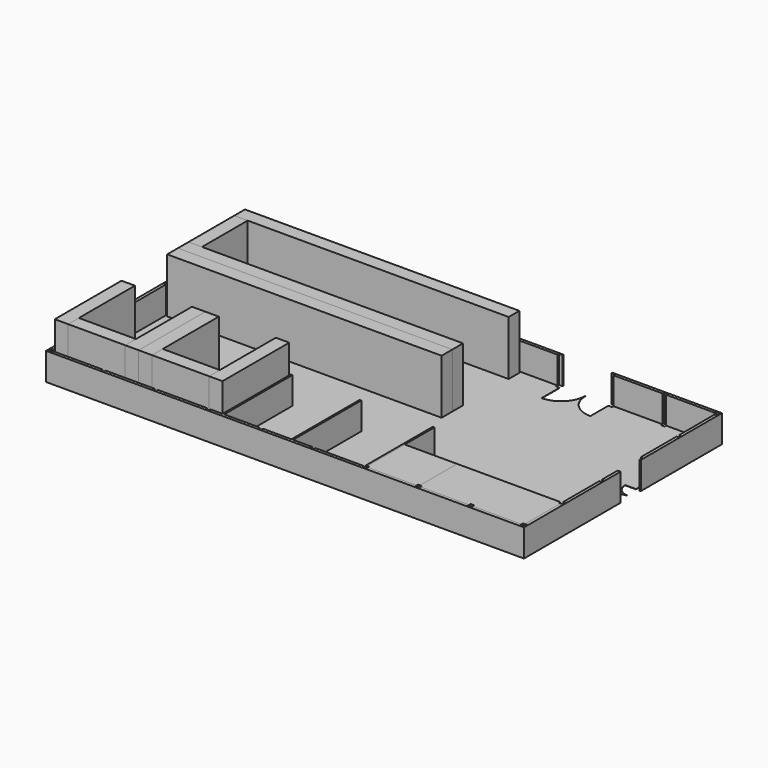
from build123d import *

# Parameters (mm, degrees)
F0_R     = 2342.0075
F0_W     = 6500
F0_H     = 150
F0_W_2   = 6127.2340836304
F1_DEPTH = 25
F2_DEPTH = 5000
F3_DEPTH = 5000
F4_DEPTH = 5000
F0_W_3   = 150
F0_H_2   = 7620
F5_DEPTH = 2500
F6_DEPTH = 2500
F7_DEPTH = 2500
F8_DEPTH = 1000
F0_H_3   = 270
F9_DEPTH = 2500


with BuildPart() as f1:
    # F0 (on Top) → F1 (new body)
    with BuildSketch(Plane.XY):
        with BuildLine():
            ThreePointArc((33274.4446, 19781.1111), (31705.4532121104, 20431.0086121104), (31055.5557, 22000))
            ThreePointArc((31055.5557, 22000), (30405.6581878896, 20431.0086121104), (28836.6668, 19781.1111))
            Line((28836.6668, 19781.1111), (28836.6668, 21830))
            Line((28836.6668, 21830), (28496.6668, 21830))
            Line((28496.6668, 21830), (28496.6668, 22000))
            Line((28496.6668, 22000), (24058.889, 22000))
            Line((24058.889, 22000), (24058.889, 21830))
            Line((24058.889, 21830), (25170, 21830))
            Line((25170, 21830), (25170, 20610))
            Line((25170, 20610), (1390, 20610))
            Line((1390, 20610), (1390, 15410))
            Line((1390, 15410), (25170, 15410))
            Line((25170, 15410), (25170, 14190))
            Line((25170, 14190), (25170, 12970))
            Line((25170, 12970), (170, 12970))
            Line((170, 12970), (170, 13030))
            Line((170, 13030), (0, 13030))
            Line((0, 13030), (0, 11370))
            Line((0, 11370), (0, 9370))
            Line((0, 9370), (0, 8970))
            Line((0, 8970), (170, 8970))
            Line((170, 8970), (170, 8630))
            Line((170, 8630), (0, 8630))
            Line((0, 8630), (0, 4570))
            Line((0, 4570), (170, 4570))
            Line((170, 4570), (170, 7770))
            Line((170, 7770), (1390, 7770))
            Line((1390, 7770), (1390, 1390))
            Line((1390, 1390), (6590, 1390))
            Line((6590, 1390), (6590, 7770))
            Line((6590, 7770), (7810, 7770))
            Line((7810, 7770), (9030, 7770))
            Line((9030, 7770), (9030, 1390))
            Line((9030, 1390), (14230, 1390))
            Line((14230, 1390), (14230, 7770))
            Line((14230, 7770), (15450, 7770))
            Line((15450, 7770), (15450, 170))
            Line((15450, 170), (14503.3334, 170))
            Line((14503.3334, 170), (14503.3334, 0))
            Line((14503.3334, 0), (15589.4327163696, 0))
            Line((15589.4327163696, 0), (15589.4327163696, 7620))
            Line((15589.4327163696, 7620), (15589.4327163696, 7770))
            Line((15589.4327163696, 7770), (15739.4327163696, 7770))
            Line((15739.4327163696, 7770), (21866.6668, 7770))
            Line((21866.6668, 7770), (22016.6668, 7770))
            Line((22016.6668, 7770), (28516.6668, 7770))
            Line((28516.6668, 7770), (28666.6668, 7770))
            Line((28666.6668, 7770), (28666.6668, 7620))
            Line((28666.6668, 7620), (28666.6668, 4400))
            Line((28666.6668, 4400), (33444.4446, 4400))
            Line((33444.4446, 4400), (42830, 4400))
            Line((42830, 4400), (42830, 4570))
            Line((42830, 4570), (43000, 4570))
            Line((43000, 4570), (43000, 8630))
            Line((43000, 8630), (42830, 8630))
            Line((42830, 8630), (42830, 8970))
            Line((42830, 8970), (43000, 8970))
            Line((43000, 8970), (43000, 10730))
            Line((43000, 10730), (41850, 10730))
            ThreePointArc((41850, 10730), (42186.8272016355, 11543.1727983645), (43000, 11880))
            ThreePointArc((43000, 11880), (42186.8272016355, 12216.8272016355), (41850, 13030))
            Line((41850, 13030), (42830, 13030))
            Line((42830, 13030), (42830, 13370))
            Line((42830, 13370), (43000, 13370))
            Line((43000, 13370), (43000, 17430))
            Line((43000, 17430), (42830, 17430))
            Line((42830, 17430), (42830, 17770))
            Line((42830, 17770), (43000, 17770))
            Line((43000, 17770), (43000, 21830))
            Line((43000, 21830), (42830.0002, 21830))
            Line((42830.0002, 21830), (42830.0002, 22000))
            Line((42830.0002, 22000), (38392.2224, 22000))
            Line((38392.2224, 22000), (38392.2224, 21830))
            Line((38392.2224, 21830), (38052.2224, 21830))
            Line((38052.2224, 21830), (38052.2224, 22000))
            Line((38052.2224, 22000), (33614.4446, 22000))
            Line((33614.4446, 22000), (33614.4446, 21830))
            Line((33614.4446, 21830), (33274.4446, 21830))
            Line((33274.4446, 21830), (33274.4446, 19781.1111))
        make_face()
        with Locations((3977.1852493286, 4560.0461959839)):
            Circle(F0_R, mode=Mode.SUBTRACT)
        with Locations((11629.6815872192, 4634.8571777344)):
            Circle(F0_R, mode=Mode.SUBTRACT)
        with Locations((5527.8644561768, 18056.058883667)):
            Circle(F0_R, mode=Mode.SUBTRACT)
        Polygon((15739.4327163696, 7620), (15739.4327163696, 0), (18941.1112, 0), (18941.1112, 170), (19281.1112, 170), (19281.1112, 0), (21866.6668, 0), (21866.6668, 7620), align=None)
        Polygon((22016.6668, 7620), (22016.6668, 0), (23718.889, 0), (23718.889, 170), (24058.889, 170), (24058.889, 0), (28496.6668, 0), (28496.6668, 170), (28516.6668, 170), (28516.6668, 7620), align=None)
        with Locations((25266.6668, 7695)):
            Rectangle(F0_W, F0_H)
        with Locations((18803.0497581848, 7695)):
            Rectangle(F0_W_2, F0_H)
    extrude(amount=F1_DEPTH)

    # F0 (on Top) → F5 (join)
    with BuildSketch(Plane.XY):
        with Locations((15664.4327163696, 3810)):
            Rectangle(F0_W_3, F0_H_2)
        with Locations((15664.4327163696, 7695)):
            Rectangle(F0_W_3, F0_H)
        with Locations((21941.6668, 7695)):
            Rectangle(F0_W_3, F0_H)
        with Locations((21941.6668, 3810)):
            Rectangle(F0_W_3, F0_H_2)
        with Locations((28591.6668, 7695)):
            Rectangle(F0_W_3, F0_H)
        Polygon((28666.6668, 7620), (28516.6668, 7620), (28516.6668, 170), (28666.6668, 170), (28666.6668, 4400), align=None)
    extrude(amount=F5_DEPTH)

    # F0 (on Top) → F9 (join)
    with BuildSketch(Plane.XY):
        Polygon((43270.0002, -270), (43270.0002, 10730), (43000, 10730), (43000, 8970), (43170, 8970), (43170, 8630), (43000, 8630), (43000, 4570), (43170, 4570), (43170, 4230), (43000.0000077273, 4230), (43000.0001922727, 170), (43170.0002, 170), (43170.0002, -170), (42830.0002, -170), (42830.0002, 0), (38392.2224, 0), (38392.2224, -170), (38052.2224, -170), (38052.2224, 0), (33614.4446, 0), (33614.4446, -170), (33274.4446, -170), (33274.4446, 0), (28836.6668, 0), (28836.6668, -170), (28516.6668, -170), (28516.6668, -270), align=None)
        Polygon((33614.4446, 22170), (33614.4446, 22000), (38052.2224, 22000), (38052.2224, 22170), (38392.2224, 22170), (38392.2224, 22000), (42830.0002, 22000), (42830.0002, 22170), (43170.0002, 22170), (43170.0002, 21830), (43000, 21830), (43000, 17770), (43170, 17770), (43170, 17430), (43000, 17430), (43000, 13370), (43170, 13370), (43170, 13030), (43270.0002, 13030), (43270.0002, 22270), (33274.4446, 22270), (33274.4446, 22170), align=None)
        Polygon((22016.6668, 0), (22016.6668, -270), (28516.6668, -270), (28516.6668, -170), (28496.6668, -170), (28496.6668, 0), (24058.889, 0), (24058.889, -170), (23718.889, -170), (23718.889, 0), align=None)
        Polygon((15739.4327163696, 0), (15739.4327163696, -270), (21866.6668, -270), (21866.6668, 0), (19281.1112, 0), (19281.1112, -170), (18941.1112, -170), (18941.1112, 0), align=None)
        with Locations((21941.6668, -135)):
            Rectangle(F0_W_3, F0_H_3)
        with Locations((15664.4327163696, -135)):
            Rectangle(F0_W_3, F0_H_3)
        Polygon((24058.889, 22000), (28496.6668, 22000), (28496.6668, 22170), (28836.6668, 22170), (28836.6668, 22270), (-270, 22270), (-270, -270), (15589.4327163696, -270), (15589.4327163696, 0), (14503.3334, 0), (14503.3334, -170), (14163.3334, -170), (14163.3334, 0), (9725.5556, 0), (9725.5556, -170), (9385.5556, -170), (9385.5556, 0), (4947.7778, 0), (4947.7778, -170), (4607.7778, -170), (4607.7778, 0), (170, 0), (170, -170), (-170, -170), (-170, 170), (0, 170), (0, 4230), (-170, 4230), (-170, 4570), (0, 4570), (0, 8630), (-170, 8630), (-170, 8970), (0, 8970), (0, 9370), (0, 11370), (0, 13030), (-170, 13030), (-170, 13370), (0, 13370), (0, 17430), (-170, 17430), (-170, 17770), (0, 17770), (0, 21830), (-170, 21830), (-170, 22170), (170, 22170), (170, 22000), (4607.7778, 22000), (4607.7778, 22170), (4947.7778, 22170), (4947.7778, 22000), (9385.5556, 22000), (9385.5556, 22170), (9725.5556, 22170), (9725.5556, 22000), (14163.3334, 22000), (14163.3334, 22170), (14503.3334, 22170), (14503.3334, 22000), (18941.1112, 22000), (18941.1112, 22170), (19281.1112, 22170), (19281.1112, 22000), (23718.889, 22000), (23718.889, 22170), (24058.889, 22170), align=None)
    extrude(amount=F9_DEPTH)


with BuildPart() as f2:
    # F0 (on Top) → F2 (new body)
    with BuildSketch(Plane.XY):
        Polygon((25170, 15410), (1390, 15410), (170, 15410), (170, 14190), (25170, 14190), align=None)
    extrude(amount=F2_DEPTH)


with BuildPart() as f2b:
    # F0 (on Top) → F2, piece 2 (new body)
    with BuildSketch(Plane.XY):
        Polygon((170, 4230), (170, 170), (1390, 170), (1390, 1390), (1390, 7770), (170, 7770), (170, 4570), align=None)
    extrude(amount=F2_DEPTH)


with BuildPart() as f2c:
    # F0 (on Top) → F2, piece 3 (new body)
    with BuildSketch(Plane.XY):
        Polygon((6590, 1390), (6590, 170), (7810, 170), (7810, 7770), (6590, 7770), align=None)
    extrude(amount=F2_DEPTH)


with BuildPart() as f2d:
    # F0 (on Top) → F2, piece 4 (new body)
    with BuildSketch(Plane.XY):
        Polygon((25170, 21830), (24058.889, 21830), (23718.889, 21830), (19281.1112, 21830), (18941.1112, 21830), (14503.3334, 21830), (14163.3334, 21830), (9725.5556, 21830), (9385.5556, 21830), (4947.7778, 21830), (4607.7778, 21830), (170, 21830), (170, 20610), (1390, 20610), (25170, 20610), align=None)
    extrude(amount=F2_DEPTH)


with BuildPart() as f2e:
    # F0 (on Top) → F2, piece 5 (new body)
    with BuildSketch(Plane.XY):
        Polygon((14230, 170), (14503.3334, 170), (15450, 170), (15450, 7770), (14230, 7770), (14230, 1390), align=None)
    extrude(amount=F2_DEPTH)


with BuildPart() as f3:
    # F0 (on Top) → F3 (new body)
    with BuildSketch(Plane.XY):
        Polygon((4607.7778, 170), (4947.7778, 170), (6590, 170), (6590, 1390), (1390, 1390), (1390, 170), align=None)
    extrude(amount=F3_DEPTH)


with BuildPart() as f3b:
    # F0 (on Top) → F3, piece 2 (new body)
    with BuildSketch(Plane.XY):
        Polygon((9030, 170), (9030, 1390), (9030, 7770), (7810, 7770), (7810, 170), align=None)
    extrude(amount=F3_DEPTH)


with BuildPart() as f3c:
    # F0 (on Top) → F3, piece 3 (new body)
    with BuildSketch(Plane.XY):
        Polygon((25170, 14190), (170, 14190), (170, 13370), (170, 13030), (170, 12970), (25170, 12970), align=None)
    extrude(amount=F3_DEPTH)


with BuildPart() as f3d:
    # F0 (on Top) → F3, piece 4 (new body)
    with BuildSketch(Plane.XY):
        Polygon((1390, 15410), (1390, 20610), (170, 20610), (170, 17770), (170, 17430), (170, 15410), align=None)
    extrude(amount=F3_DEPTH)


with BuildPart() as f4:
    # F0 (on Top) → F4 (new body)
    with BuildSketch(Plane.XY):
        Polygon((9725.5556, 170), (14163.3334, 170), (14230, 170), (14230, 1390), (9030, 1390), (9030, 170), (9385.5556, 170), align=None)
    extrude(amount=F4_DEPTH)


with BuildPart() as f6:
    # F0 (on Top) → F6 (new body)
    with BuildSketch(Plane.XY):
        Polygon((28836.6668, 170), (28836.6668, 0), (33274.4446, 0), (33274.4446, 170), (33444.4446, 170), (33444.4446, 4400), (28666.6668, 4400), (28666.6668, 170), align=None)
    extrude(amount=F6_DEPTH)


with BuildPart() as f7:
    # F0 (on Top) → F7 (new body)
    with BuildSketch(Plane.XY):
        Polygon((43000.0001922727, 170), (43000.0000077273, 4230), (42830, 4230), (42830, 4400), (33444.4446, 4400), (33444.4446, 170), (33614.4446, 170), (33614.4446, 0), (38052.2224, 0), (38052.2224, 170), (38392.2224, 170), (38392.2224, 0), (42830.0002, 0), (42830.0002, 170), align=None)
    extrude(amount=F7_DEPTH)


with BuildPart() as f8:
    # F0 (on Top) → F8 (new body)
    with BuildSketch(Plane.XY):
        with Locations((5527.8644561768, 18056.058883667)):
            Circle(F0_R)
    extrude(amount=F8_DEPTH)


with BuildPart() as f8b:
    # F0 (on Top) → F8, piece 2 (new body)
    with BuildSketch(Plane.XY):
        with Locations((3977.1852493286, 4560.0461959839)):
            Circle(F0_R)
    extrude(amount=F8_DEPTH)


with BuildPart() as f8c:
    # F0 (on Top) → F8, piece 3 (new body)
    with BuildSketch(Plane.XY):
        with Locations((11629.6815872192, 4634.8571777344)):
            Circle(F0_R)
    extrude(amount=F8_DEPTH)


solid = Compound([f1.part, f2.part, f2b.part, f2c.part, f2d.part, f2e.part, f3.part, f3b.part, f3c.part, f3d.part, f4.part, f6.part, f7.part, f8.part, f8b.part, f8c.part])
